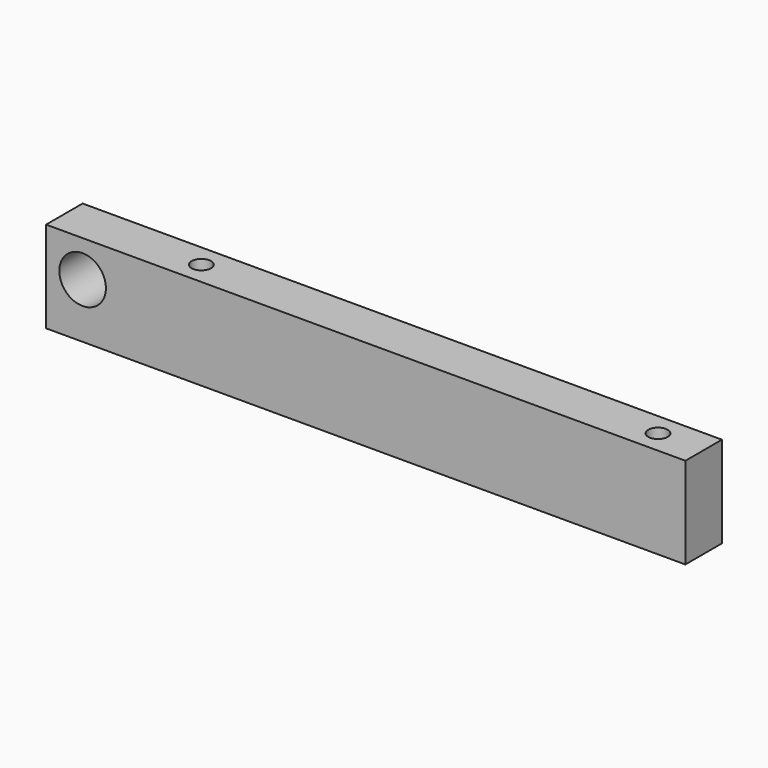
from build123d import *

# Parameters (mm, degrees)
F0_W     = 88.9
F0_H     = 12.7
F0_R     = 3.2385
F1_DEPTH = 6.35
F3_D     = 2.7051


with BuildPart() as f1:
    # F0 (on Front) → F1 (new body)
    with BuildSketch(Plane.XZ):
        Rectangle(F0_W, F0_H)
        with Locations((-39.37, 1.27)):
            Circle(F0_R, mode=Mode.SUBTRACT)
    extrude(amount=F1_DEPTH)

    # F3 (through all)
    with Locations(Plane(origin=(0, 0, -6.35), x_dir=(1, 0, 0), z_dir=(0, 0, -1))):
        with Locations((-25.4, 3.175), (38.1, 3.175)):
            Hole(F3_D / 2)


solid = f1.part
